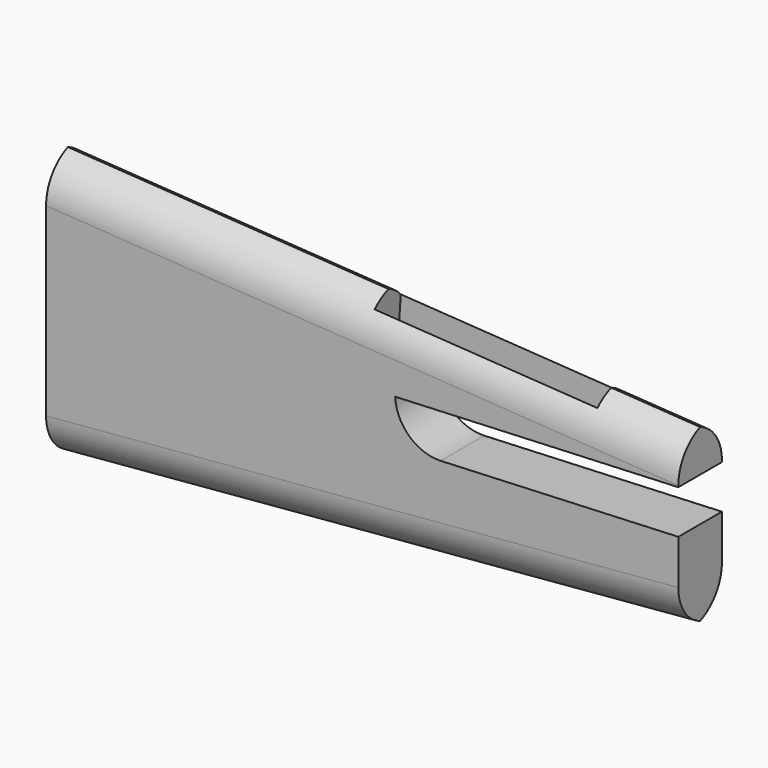
from build123d import *

# Parameters (mm, degrees)
F1_DEPTH    = 6.35
F2_W        = 3.81
F2_H        = 19.05
F3_DEPTH    = 7.62
F4_R        = 1.27
F5_R        = 1.27
F7_DEPTH    = 5.08
F8_T1_DEPTH = 99.3332002554
F8_T3_DEPTH = 99.2137995652
F9_R        = 5.07999


# Not quite as in the source:
# - a fillet or chamfer that OpenCascade refuses, or shapes differently, is made with other operations: its cross-section is extruded or revolved along the edge and cut away or added
# - a fillet or chamfer is up to 0.001 mm smaller than in the source, because OpenCascade refuses the exact size


with BuildPart() as f1:
    # F0 (on Front) → F1 (new body)
    with BuildSketch(Plane.XZ):
        Polygon((28.8813739334, 7.6191808492), (28.8813739334, 12.8777329371), (-44.7786260666, 17.6402329371), (-44.7786260666, -14.1097670629), (28.8813739334, -7.7597670629), (28.8813739334, 2.5343412086), (-3.8856118554, 1.1037037128), (-4.1071983432, 6.1788686784), align=None)
    extrude(amount=F1_DEPTH)

    # F2 (on face) → F3 (cut)
    with BuildSketch(Plane(origin=(-44.7786260666, 0, 0), x_dir=(0, -1, 0), z_dir=(-1, 0, 0))):
        with Locations((3.175, 1.7652329371)):
            Rectangle(F2_W, F2_H)
    extrude(amount=-F3_DEPTH, mode=Mode.SUBTRACT)

    # F4
    f4_edges = [f1.edges().sort_by_distance(p)[0] for p in [
        (-37.158626, -3.175, -7.759767),
    ]]
    fillet(f4_edges, radius=F4_R)

    # F5
    f5_edges = [f1.edges().sort_by_distance(p)[0] for p in [
        (-37.158626, -3.175, 11.290233),
        (-37.158626, -5.08, 2.400233),
        (-37.158626, -1.27, 2.400233),
    ]]
    fillet(f5_edges, radius=F5_R)

    # F6 (on face) → F7 (cut)
    with BuildSketch(Plane(origin=(0.9493759321, 0, 14.6836810837), x_dir=(0.9979163847, 0, -0.0645204559), z_dir=(0.0645204559, 0, 0.9979163847))):
        Polygon((15.2903190595, -1.27), (2.5903190595, -1.27), (-8.3756055683, -1.27), (-8.3756055683, -5.08), (15.2903190595, -5.08), (17.6343005151, -5.08), (17.6343005151, -1.27), align=None)
    extrude(amount=-F7_DEPTH, mode=Mode.SUBTRACT)

    # F8: fillet of radius 5.08 on 4 edges, made by hand

    # F8_s2 → F8_t1 (cut)
    with BuildSketch(Plane(origin=(-58.308759718, 0, -5.0266172171), x_dir=(0, 1, 0), z_dir=(0.996304769, 0, 0.0858883422))):
        with BuildLine():
            ThreePointArc((-6.35, -5.1316662572), (-4.8621024484, -8.7237687056), (-1.27, -10.2116662572))
            Line((-1.27, -10.2116662572), (-6.35, -10.2116662572))
            Line((-6.35, -10.2116662572), (-6.35, -5.1316662572))
        make_face()
        with BuildLine():
            ThreePointArc((0, -5.1316662572), (-1.4878975516, -8.7237687056), (-5.08, -10.2116662572))
            Line((-5.08, -10.2116662572), (0, -10.2116662572))
            Line((0, -10.2116662572), (0, -5.1316662572))
        make_face()
    extrude(amount=F8_T1_DEPTH, mode=Mode.SUBTRACT)

    # F8_s4 → F8_t3 (cut)
    with BuildSketch(Plane(origin=(40.6055360865, 0, -2.6253579366), x_dir=(0, 1, 0), z_dir=(-0.9979163847, 0, 0.0645204559))):
        with BuildLine():
            ThreePointArc((-1.27, -14.7143401085), (-4.8621024484, -13.2264425569), (-6.35, -9.6343401085))
            Line((-6.35, -9.6343401085), (-6.35, -14.7143401085))
            Line((-6.35, -14.7143401085), (-1.27, -14.7143401085))
        make_face()
        with BuildLine():
            ThreePointArc((-5.08, -14.7143401085), (-1.4878975516, -13.2264425569), (0, -9.6343401085))
            Line((0, -9.6343401085), (0, -14.7143401085))
            Line((0, -14.7143401085), (-5.08, -14.7143401085))
        make_face()
    extrude(amount=F8_T3_DEPTH, mode=Mode.SUBTRACT)

    # F9 (radius 5.08 in the source; OpenCascade refuses exactly that, so slightly less here)
    f9_edges = [f1.edges().sort_by_distance(p)[0] for p in [
        (-3.885612, -3.175, 1.103704),
    ]]
    fillet(f9_edges, radius=F9_R)


solid = f1.part
